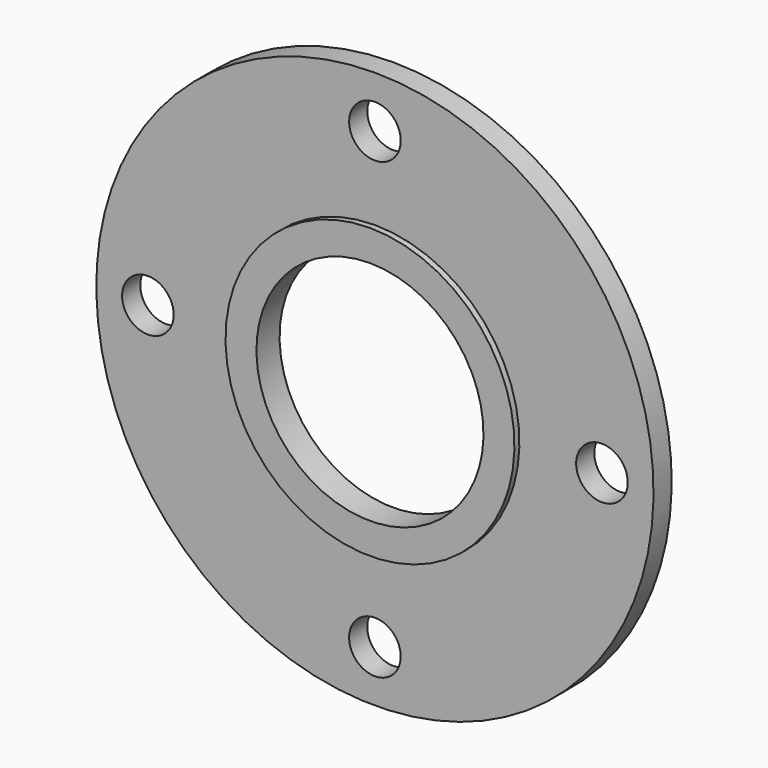
from build123d import *

# Parameters (mm, degrees)
F3_D            = 25
F3_COPIES_COUNT = 4


# Not quite as in the source:
# - a pattern or mirror of a feature is missing from the dataset's text; its kind, count and spacing are read off the source's solid


with BuildPart() as f1:
    # F0 (on Right) → F1 (revolve)
    with BuildSketch(Plane.YZ):
        Polygon((0, 70), (0, 55), (14, 55), (14, 135), (3, 135), (3, 70), align=None)
    revolve(axis=Axis((0, 31.8317301571, 0), (0, 1, 0)))

    # F3 (through all)
    with Locations(Plane.XZ.offset(-3)):
        with Locations((0, 110)):
            f3 = Hole(F3_D / 2)

    # F3_copies: F3 ×4 about axis
    f3_copies_axis = Axis((0, 0, 0), (0, 1, 0))
    for i in range(1, F3_COPIES_COUNT):
        add(f3.rotate(f3_copies_axis, i * 360 / F3_COPIES_COUNT), mode=Mode.SUBTRACT)


solid = f1.part
